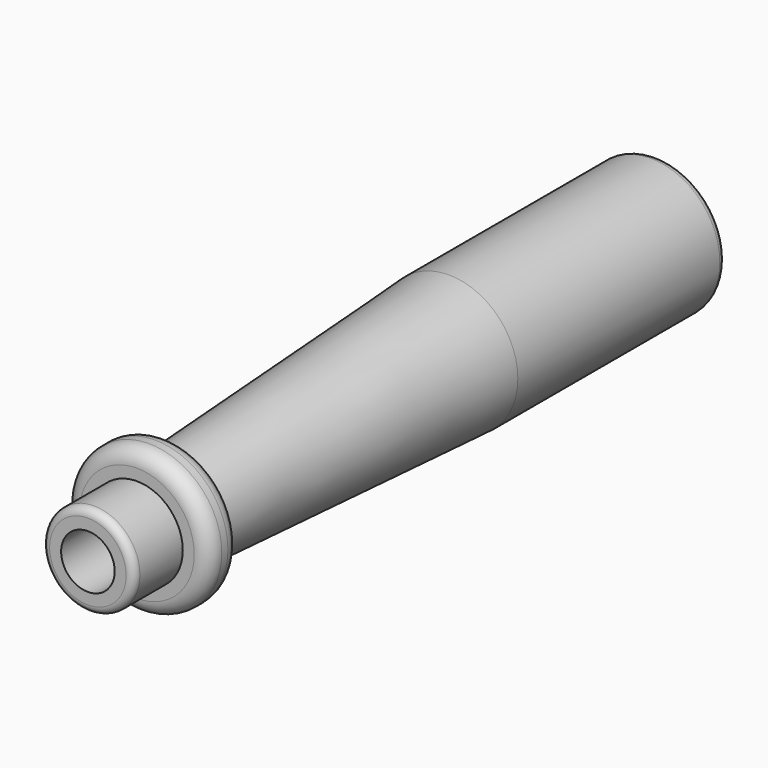
from build123d import *

# Parameters (mm, degrees)
F0_R      = 9
F1_DEPTH  = 34
F2_R      = 9
F4_R      = 6.5
F6_R      = 9.5
F7_DEPTH  = 5
F8_R      = 2
F9_R      = 6
F10_DEPTH = 8
F11_R     = 6
F12_DEPTH = 36.5
F13_R     = 7
F13_R_2   = 6
F14_DEPTH = 1.5
F15_R     = 1
F16_R     = 0.49999
F17_R     = 3.5
F18_DEPTH = 25
F19_R     = 1
F20_R     = 3.25
F20_R_2   = 3
F21_DEPTH = 11


# Not quite as in the source:
# - a fillet or chamfer is up to 0.001 mm smaller than in the source, because OpenCascade refuses the exact size


with BuildPart() as f1:
    # F0 (on Front) → F1 (new body)
    with BuildSketch(Plane.XZ):
        Circle(F0_R)
    extrude(amount=F1_DEPTH)

    # F2 (on face) → F5 section 0
    with BuildSketch(Plane.XZ.offset(34)):
        Circle(F2_R)
    # F4 (on offset) → F5 section 1
    with BuildSketch(Plane.XZ.offset(80)):
        Circle(F4_R)
    loft()

    # F6 (on face) → F7 (join)
    with BuildSketch(Plane.XZ.offset(80)):
        Circle(F6_R)
    extrude(amount=F7_DEPTH)

    # F8
    f8_edges = [f1.edges().sort_by_distance(p)[0] for p in [
        (-9.5, -85, 0),
        (-9.5, -80, 0),
    ]]
    fillet(f8_edges, radius=F8_R)

    # F9 (on face) → F10 (join)
    with BuildSketch(Plane.XZ.offset(85)):
        Circle(F9_R)
    extrude(amount=F10_DEPTH)

    # F11 (on face) → F12 (cut)
    with BuildSketch(Plane(origin=(0, 0, 0), x_dir=(-1, 0, 0), z_dir=(0, 1, 0))):
        Circle(F11_R)
    extrude(amount=-F12_DEPTH, mode=Mode.SUBTRACT)

    # F13 (on face) → F14 (join)
    with BuildSketch(Plane(origin=(0, 0, 0), x_dir=(-1, 0, 0), z_dir=(0, 1, 0))):
        Circle(F13_R)
        Circle(F13_R_2, mode=Mode.SUBTRACT)
    extrude(amount=F14_DEPTH)

    # F15
    f15_edges = [f1.edges().sort_by_distance(p)[0] for p in [
        (-9, 0, 0),
    ]]
    fillet(f15_edges, radius=F15_R)

    # F16 (radius 0.5 in the source; OpenCascade refuses exactly that, so slightly less here)
    f16_edges = [f1.edges().sort_by_distance(p)[0] for p in [
        (6, 1.5, 0),
        (7, 1.5, 0),
    ]]
    fillet(f16_edges, radius=F16_R)

    # F17 (on face) → F18 (cut)
    with BuildSketch(Plane.XZ.offset(93)):
        Circle(F17_R)
    extrude(amount=-F18_DEPTH, mode=Mode.SUBTRACT)

    # F19
    f19_edges = [f1.edges().sort_by_distance(p)[0] for p in [
        (-6, -93, 0),
    ]]
    fillet(f19_edges, radius=F19_R)

    # F20 (on face) → F21 (join)
    with BuildSketch(Plane(origin=(0, -36.5, 0), x_dir=(-1, 0, 0), z_dir=(0, 1, 0))):
        Circle(F20_R)
        Circle(F20_R_2, mode=Mode.SUBTRACT)
    extrude(amount=F21_DEPTH)


solid = f1.part
